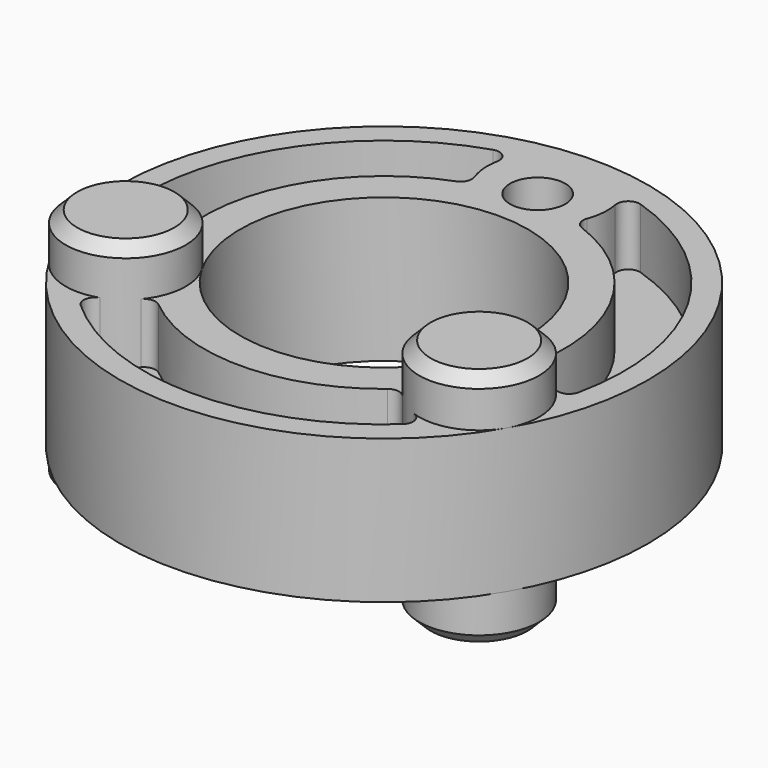
from build123d import *

# Parameters (mm, degrees)
F0_R            = 17.4625
F0_R_2          = 9.525
F0_R_3          = 1.8288
F1_DEPTH        = 9.525
F3_DEPTH        = 3.96875
F3_COPIES_COUNT = 3
F5_DEPTH        = 3.96875
F5_COPIES_COUNT = 3
F6_R            = 0.762
F8_R            = 3.96875
F9_DEPTH        = 3.175
F9_DEPTH_BACK   = 12.7
F10_SIZE        = 0.762


# Not quite as in the source:
# - a feature of the source that left no trace in its solid (it failed there, or was rolled back) is left out
# - a pattern or mirror of a feature is missing from the dataset's text; its kind, count and spacing are read off the source's solid


with BuildPart() as f1:
    # F0 (on Top) → F1 (new body)
    with BuildSketch(Plane.XY):
        Circle(F0_R)
        Circle(F0_R_2, mode=Mode.SUBTRACT)
        with Locations((0, 12.7)):
            Circle(F0_R_3, mode=Mode.SUBTRACT)
    extrude(amount=F1_DEPTH)

    # F2 (on face) → F3 (cut)
    with BuildSketch(Plane.XY.offset(9.525)):
        with BuildLine():
            ThreePointArc((-3.3814051731, 11.4159926471), (-3.9685398143, 13.4529051128), (-3.4234536074, 15.5014705882))
            ThreePointArc((-3.4234536074, 15.5014705882), (-13.7481532851, 7.9375), (-15.1363941291, -4.7859375014))
            ThreePointArc((-15.1363941291, -4.7859375014), (-13.6348274895, -3.2895962613), (-11.5772422283, -2.7796135431))
            ThreePointArc((-11.5772422283, -2.7796135431), (-10.3111149638, 5.953125), (-3.3814051731, 11.4159926471))
        make_face()
    f3 = extrude(amount=-F3_DEPTH, mode=Mode.SUBTRACT)

    # F3_copies: F3 ×3 about axis
    f3_copies_axis = Axis((0, 0, 0), (0, 0, 1))
    for i in range(1, F3_COPIES_COUNT):
        add(f3.rotate(f3_copies_axis, i * 360 / F3_COPIES_COUNT), mode=Mode.SUBTRACT)

    # F4 (on face) → F5 (cut)
    with BuildSketch(Plane(origin=(0, 0, 0), x_dir=(1, 0, 0), z_dir=(0, 0, -1))):
        with BuildLine():
            ThreePointArc((-11.5772422283, 2.7796135431), (-13.6348274895, 3.2895962613), (-15.1363941291, 4.7859375014))
            ThreePointArc((-15.1363941291, 4.7859375014), (-13.7481532851, -7.9375), (-3.4234536074, -15.5014705882))
            ThreePointArc((-3.4234536074, -15.5014705882), (-3.9685398143, -13.4529051128), (-3.3814051731, -11.4159926471))
            ThreePointArc((-3.3814051731, -11.4159926471), (-10.3111149638, -5.953125), (-11.5772422283, 2.7796135431))
        make_face()
    f5 = extrude(amount=-F5_DEPTH, mode=Mode.SUBTRACT)

    # F5_copies: F5 ×3 about axis
    f5_copies_axis = Axis((0, 0, 0), (0, 0, 1))
    for i in range(1, F5_COPIES_COUNT):
        add(f5.rotate(f5_copies_axis, i * 360 / F5_COPIES_COUNT), mode=Mode.SUBTRACT)

    # F6
    f6_edges = [f1.edges().sort_by_distance(p)[0] for p in [
        (-15.136394, -4.785938, 7.540625),
        (-11.577242, -2.779614, 7.540625),
        (-3.381405, 11.415993, 7.540625),
        (-3.423454, 15.501471, 7.540625),
        (-3.381405, 11.415993, 1.984375),
        (-3.423454, 15.501471, 1.984375),
        (-11.577242, -2.779614, 1.984375),
        (-15.136394, -4.785938, 1.984375),
        (8.195837, -8.636379, 1.984375),
        (11.712941, -10.715533, 1.984375),
        (-8.195837, -8.636379, 1.984375),
        (-11.712941, -10.715533, 1.984375),
        (3.381405, 11.415993, 1.984375),
        (3.423454, 15.501471, 1.984375),
        (11.577242, -2.779614, 1.984375),
        (15.136394, -4.785938, 1.984375),
        (11.712941, -10.715533, 7.540625),
        (8.195837, -8.636379, 7.540625),
        (-11.712941, -10.715533, 7.540625),
        (-8.195837, -8.636379, 7.540625),
        (3.423454, 15.501471, 7.540625),
        (3.381405, 11.415993, 7.540625),
        (11.577242, -2.779614, 7.540625),
        (15.136394, -4.785938, 7.540625),
    ]]
    fillet(f6_edges, radius=F6_R)

    # F8 (on face) → F9 (join, two sides)
    with BuildSketch(Plane(origin=(0, 0, 0), x_dir=(1, 0, 0), z_dir=(0, 0, -1))) as f9_sk:
        with Locations((11.6859302923, 6.746875)):
            Circle(F8_R)
        with Locations((-11.6859302923, 6.746875)):
            Circle(F8_R)
    extrude(amount=F9_DEPTH)
    extrude(f9_sk.sketch, amount=-F9_DEPTH_BACK)

    # F10
    f10_edges = [f1.edges().sort_by_distance(p)[0] for p in [
        (-15.65468, -6.746875, 12.7),
        (7.71718, -6.746875, 12.7),
        (7.71718, -6.746875, -3.175),
        (-15.65468, -6.746875, -3.175),
    ]]
    chamfer(f10_edges, length=F10_SIZE)


solid = f1.part
